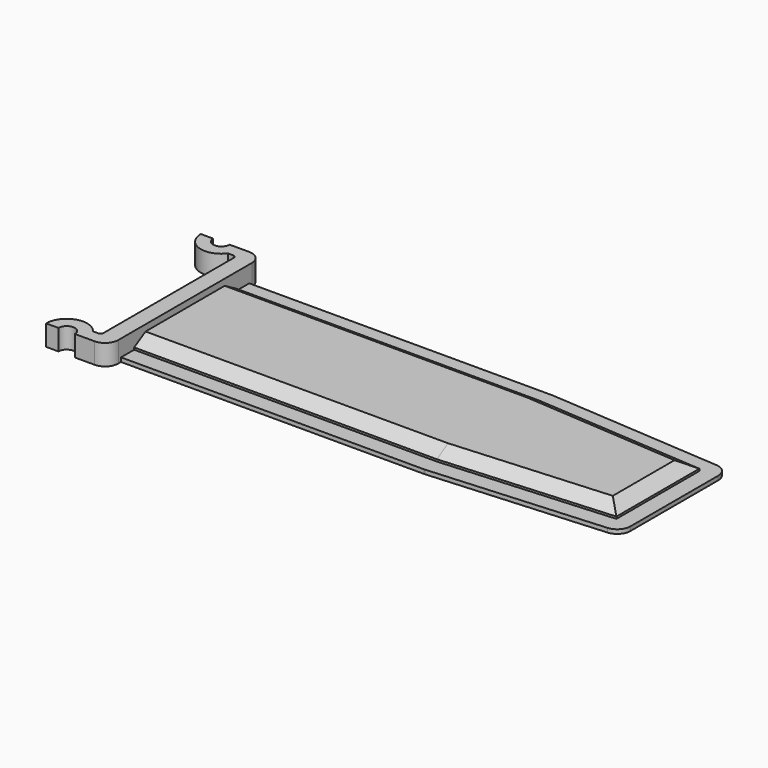
from build123d import *

# Parameters (mm, degrees)
F1_DEPTH    = 2.125
F3_DEPTH    = 1.5875
F5_DEPTH    = 0.79375
F7_DEPTH    = 3.175
F7_TAPER    = 60
F8_T1_DEPTH = 25.2718606601
F8_T3_DEPTH = 2.4753029305
F9_W        = 5.499261314
F9_H        = 61.9125
F10_DEPTH   = 3.96875
F11_W       = 31.75
F11_H       = 4.25
F12_DEPTH   = 2.38125
F14_DEPTH   = 8
F15_W       = 36.5125
F15_H       = 2.38125
F16_DEPTH   = 25.4
F17_R       = 5.08
F18_R       = 1.27


# Not quite as in the source:
# - a fillet or chamfer that OpenCascade refuses, or shapes differently, is made with other operations: its cross-section is extruded or revolved along the edge and cut away or added


with BuildPart() as f1:
    # F0 (on Top) → F1 (new body, symmetric)
    with BuildSketch(Plane.XY):
        Polygon((31.75, 15.875), (-88.9, 15.875), (-88.9, -15.875), (31.75, -15.875), (88.9, -11.875), (88.9, 11.875), align=None)
    extrude(amount=F1_DEPTH, both=True)

    # F11 (on face) → F12 (join, through all)
    with BuildSketch(Plane(origin=(-88.9, 0, 0), x_dir=(0, -1, 0), z_dir=(-1, 0, 0))):
        Rectangle(F11_W, F11_H)
    extrude(amount=F12_DEPTH)


with BuildPart() as f3:
    # F2 (on Top) → F3 (new body)
    with BuildSketch(Plane.XY):
        Polygon((-91.28125, 18.25625), (31.8332315247, 18.25625), (91.28125, 14.0954088119), (91.28125, -14.0954088119), (31.8332315247, -18.25625), (-91.28125, -18.25625), (-91.28125, -30.95625), (32.27713299, -30.95625), (103.98125, -25.9375891419), (103.98125, 25.9375891419), (32.27713299, 30.95625), (-91.28125, 30.95625), align=None)
    extrude(amount=F3_DEPTH)

    # F4 (on face) → F5 (join)
    with BuildSketch(Plane.XY.offset(1.5875)):
        Polygon((91.28125, -14.0954088119), (31.8332315247, -18.25625), (-91.28125, -18.25625), (-91.28125, -24.60625), (32.0551822574, -24.60625), (97.63125, -20.0164989769), (97.63125, 20.0164989769), (32.0551822574, 24.60625), (-91.28125, 24.60625), (-91.28125, 18.25625), (31.8332315247, 18.25625), (91.28125, 14.0954088119), align=None)
    extrude(amount=F5_DEPTH)

    # F6 (on face) → F7 (join)
    with BuildSketch(Plane.XY.offset(2.38125)):
        Polygon((-91.28125, 24.60625), (-91.28125, -24.60625), (32.0551822574, -24.60625), (97.63125, -20.0164989769), (97.63125, 20.0164989769), (32.0551822574, 24.60625), align=None)
    extrude(amount=F7_DEPTH, taper=F7_TAPER)

    # F8: fillet of radius 5.08 on 4 edges, made by hand

    # F8_s2 → F8_t1 (cut)
    with BuildSketch(Plane.XY.offset(-11.84218033)):
        with BuildLine():
            ThreePointArc((103.98125, -21.2007170099), (102.616637885, -24.6651495556), (99.2559378489, -26.2683196512))
            Line((99.2559378489, -26.2683196512), (103.98125, -25.9375891419))
            Line((103.98125, -25.9375891419), (103.98125, -21.2007170099))
        make_face()
        with BuildLine():
            ThreePointArc((99.2559378489, 26.2683196512), (102.616637885, 24.6651495556), (103.98125, 21.2007170099))
            Line((103.98125, 21.2007170099), (103.98125, 25.9375891419))
            Line((103.98125, 25.9375891419), (99.2559378489, 26.2683196512))
        make_face()
    extrude(amount=F8_T1_DEPTH, mode=Mode.SUBTRACT)

    # F8_s4 → F8_t3 (cut)
    with BuildSketch(Plane.XY.offset(-0.4439014652)):
        with BuildLine():
            ThreePointArc((32.0995724039, -30.95625), (32.2770246261, -30.9531497143), (32.4542602528, -30.9438526413))
            Line((32.4542602528, -30.9438526413), (32.27713299, -30.95625))
            Line((32.27713299, -30.95625), (32.0995724039, -30.95625))
        make_face()
        with BuildLine():
            ThreePointArc((32.0995724039, 30.95625), (32.2770246261, 30.9531497143), (32.4542602528, 30.9438526413))
            Line((32.4542602528, 30.9438526413), (32.27713299, 30.95625))
            Line((32.27713299, 30.95625), (32.0995724039, 30.95625))
        make_face()
    extrude(amount=F8_T3_DEPTH, mode=Mode.SUBTRACT)

    # F9 (on face) → F10 (join, through all)
    with BuildSketch(Plane.XY.offset(1.5875)):
        with Locations((-88.531619343, 0)):
            Rectangle(F9_W, F9_H)
    extrude(amount=F10_DEPTH)

    # F13 (on Top) → F14 (join)
    with BuildSketch(Plane.XY):
        with BuildLine():
            Line((-103.98125, 37.35), (-108.74375, 37.35))
            ThreePointArc((-108.74375, 37.35), (-103.3163078928, 29.8198263217), (-94.45625, 32.5875))
            Line((-94.45625, 32.5875), (-91.28125, 32.5875))
            Line((-91.28125, 32.5875), (-91.28125, 0))
            Line((-91.28125, 0), (-91.28125, -32.5875))
            Line((-91.28125, -32.5875), (-94.45625, -32.5875))
            ThreePointArc((-94.45625, -32.5875), (-103.3163078928, -29.8198263217), (-108.74375, -37.35))
            Line((-108.74375, -37.35), (-103.98125, -37.35))
            ThreePointArc((-103.98125, -37.35), (-100.80625, -34.175), (-97.63125, -37.35))
            Line((-97.63125, -37.35), (-84.93125, -37.35))
            Line((-84.93125, -37.35), (-84.93125, 0))
            Line((-84.93125, 0), (-84.93125, 37.35))
            Line((-84.93125, 37.35), (-97.63125, 37.35))
            ThreePointArc((-97.63125, 37.35), (-100.80625, 34.175), (-103.98125, 37.35))
        make_face()
    extrude(amount=F14_DEPTH)

    # F15 (on face) → F16 (cut)
    with BuildSketch(Plane(origin=(-91.28125, 0, 0), x_dir=(0, -1, 0), z_dir=(-1, 0, 0))):
        with Locations((0, 1.190625)):
            Rectangle(F15_W, F15_H)
    extrude(amount=-F16_DEPTH, mode=Mode.SUBTRACT)

    # F17
    f17_edges = [f3.edges().sort_by_distance(p)[0] for p in [
        (-84.93125, 37.35, 4),
        (-84.93125, -37.35, 4),
    ]]
    fillet(f17_edges, radius=F17_R)

    # F18
    f18_edges = [f3.edges().sort_by_distance(p)[0] for p in [
        (-91.28125, -32.5875, 4),
        (-91.28125, 32.5875, 4),
    ]]
    fillet(f18_edges, radius=F18_R)


solid = Compound([f1.part, f3.part])
